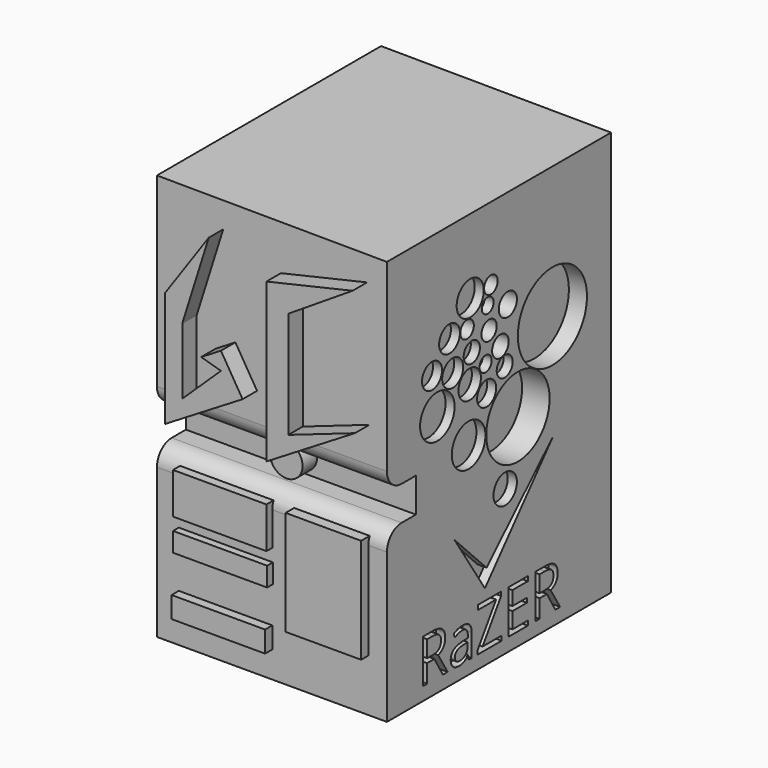
from build123d import *

# Parameters (mm, degrees)
F1_DEPTH      = 77.47
F3_DEPTH      = 5
F4_W          = 25.8451560512
F4_H          = 11.3645372912
F4_W_2        = 26.0284543037
F4_H_2        = 5.3156707436
F5_DEPTH      = 2
F6_R          = 2.3473696574
F7_DEPTH      = 10
F8_R          = 2.3473719846
F9_DEPTH      = 5
F10_R         = 2.6437582776
F11_DEPTH     = 5
F12_R         = 3.137573147
F13_DEPTH     = 5
F14_R         = 2.8690843811
F15_DEPTH     = 5
F16_R         = 11.9496313733
F17_DEPTH     = 5
F18_R         = 10.9566184267
F19_DEPTH     = 7.62
F20_W         = 59.5721621066
F20_H         = 108.5129901767
F21_DEPTH     = 0.5
F22_W         = 17.9633004591
F22_H         = 7.5152590871
F22_W_2       = 17.7800012752
F22_H_2       = 5.4989699274
F22_W_3       = 4.9490742385
F22_H_3       = 2.7494849637
F22_W_4       = 23.4622657299
F22_H_4       = 5.1323715597
F22_W_5       = 23.0956692249
F22_H_5       = 5.3156688809
F22_W_6       = 5.1323715597
F22_W_7       = 5.1323659718
F23_DEPTH     = 4
F24_TEXT_SIZE = 26.2153474792
F25_DEPTH     = 8.382
F26_R         = 6.3549509032
F27_DEPTH     = 6.604
F28_W         = 25.8451560512
F28_H         = 5.8655701578
F28_W_2       = 20.8960818127
F28_H_2       = 28.9612365887
F29_DEPTH     = 2.5
F30_R         = 3.6383810655
F30_R_2       = 3.8883576081
F30_R_3       = 3.3044699567
F30_R_4       = 2.0493435113
F30_R_5       = 2.8039346928
F30_R_6       = 2.0899281645
F30_R_7       = 5.8253336684
F30_R_8       = 5.967781049
F30_R_9       = 2.7494855225
F30_R_10      = 4.6839974373
F30_R_11      = 3.6012530141
F30_R_12      = 3.4584789248
F31_DEPTH     = 2.5
F32_W         = 18.5131970793
F32_H         = 58.8389690965
F33_DEPTH     = 1.5
F34_W         = 15.5804110691
F34_H         = 5.4989689961
F34_W_2       = 4.0325764567
F34_H_2       = 7.8818553593
F34_H_3       = 8.065154776
F34_W_3       = 4.4908244163
F34_W_4       = 15.2138136327
F34_H_4       = 5.6822672486
F35_DEPTH     = 5.588
F36_R         = 3.3044699309
F37_DEPTH     = 4.318
F38_W         = 63.6047441512
F38_H         = 9.4942739233
F39_DEPTH     = 10
F40_T1_DEPTH  = 18.9321648002
F40_T6_DEPTH  = 28.0447434634
F40_T11_DEPTH = 42.0278358877
F40_T16_DEPTH = 89.0047441512
F40_T21_DEPTH = 89.0047441512
F40_T26_DEPTH = 89.0047441512
F40_T32_DEPTH = 89.0047441512
F41_R         = 4.4746184375
F42_DEPTH     = 5
F43_R         = 4.0432169308
F44_DEPTH     = 2.54
F45_TEXT_SIZE = 16.8991896013
F46_DEPTH     = 2.5


# Not quite as in the source:
# - a fillet or chamfer that OpenCascade refuses, or shapes differently, is made with other operations: its cross-section is extruded or revolved along the edge and cut away or added
# - Text() gives the source's letters only with a copy of the font that has no kerning and outlines rounded to 1/6400 em; it was checked with that copy


with BuildPart() as f1:
    # F0 (on Front) → F1 (new body)
    with BuildSketch(Plane.XZ):
        Polygon((18.4215474874, 56.0894832015), (-45.1831966639, 56.4560852945), (-45.1831966639, -55.9061877429), (18.4215474874, -55.9061877429), align=None)
    extrude(amount=F1_DEPTH)

    # F2 (on face) → F3 (join)
    with BuildSketch(Plane.XZ.offset(77.47)):
        Polygon((-34.1852605343, 26.0284524411), (-26.8532987684, 49.3074245751), (-38.9510318637, 31.8940207362), (-38.9510318637, 0), (-17.5050515682, 13.0142262205), (-23.4882612947, 22.8738825479), (-28.9533808628, 19.5574427582), (-23.4882612947, 17.9632995278), (-34.1852605343, 7.6985568739), align=None)
        Polygon((-4.8574223183, 37.9428863525), (12.9225775599, 49.3074245751), (-10.9062884003, 43.808452785), (-10.9062884003, 0), (13.5728147639, 14.8548390824), (-4.8574223183, 8.4317522123), align=None)
    extrude(amount=F3_DEPTH)

    # F4 (on face) → F5 (join)
    with BuildSketch(Plane.XZ.offset(77.47)):
        with Locations((-26.2117530219, -18.1465991773)):
            Rectangle(F4_W, F4_H)
        with Locations((-26.1201038957, -29.9693820998)):
            Rectangle(F4_W_2, F4_H_2)
    extrude(amount=F5_DEPTH)

    # F6 (on face) → F7 (cut)
    with BuildSketch(Plane.YZ.offset(18.4215474874)):
        with Locations((-41.5361337364, 35.9265990555)):
            Circle(F6_R)
    extrude(amount=-F7_DEPTH, mode=Mode.SUBTRACT)

    # F8 (on face) → F9 (cut, symmetric)
    with BuildSketch(Plane.YZ.offset(18.4215474874)):
        with Locations((-49.7845895588, 28.4113399684)):
            Circle(F8_R)
    extrude(amount=F9_DEPTH, both=True, mode=Mode.SUBTRACT)

    # F10 (on face) → F11 (cut, symmetric)
    with BuildSketch(Plane.YZ.offset(18.4215474874)):
        with Locations((-42.1596653759, 25.0808000565)):
            Circle(F10_R)
    extrude(amount=F11_DEPTH, both=True, mode=Mode.SUBTRACT)

    # F12 (on face) → F13 (cut, symmetric)
    with BuildSketch(Plane.YZ.offset(18.4215474874)):
        with Locations((-35.6705673039, 28.7779401988)):
            Circle(F12_R)
    extrude(amount=F13_DEPTH, both=True, mode=Mode.SUBTRACT)

    # F14 (on face) → F15 (cut, symmetric)
    with BuildSketch(Plane.YZ.offset(18.4215474874)):
        with Locations((-38.2367521524, 19.6129903197)):
            Circle(F14_R)
    extrude(amount=F15_DEPTH, both=True, mode=Mode.SUBTRACT)

    # F16 (on face) → F17 (cut, symmetric)
    with BuildSketch(Plane.YZ.offset(18.4215474874)):
        with Locations((-20.2734526247, 19.6129903197)):
            Circle(F16_R)
    extrude(amount=F17_DEPTH, both=True, mode=Mode.SUBTRACT)

    # F18 (on face) → F19 (cut, symmetric)
    with BuildSketch(Plane.YZ.offset(18.4215474874)):
        with Locations((-32.1878865361, 0)):
            Circle(F18_R)
    extrude(amount=F19_DEPTH, both=True, mode=Mode.SUBTRACT)

    # F20 (on face) → F21 (cut, symmetric)
    with BuildSketch(Plane.XZ):
        with Locations((-13.5641237721, 0.1832991838)):
            Rectangle(F20_W, F20_H)
    extrude(amount=F21_DEPTH, both=True, mode=Mode.SUBTRACT)

    # F22 (on face) → F23 (cut, symmetric)
    with BuildSketch(Plane.XZ):
        with Locations((2.84113409, 43.9001061022)):
            Rectangle(F22_W, F22_H)
        with Locations((2.7494844981, 26.7616501078)):
            Rectangle(F22_W_2, F22_H_2)
        with Locations((-20.1628860086, 7.2403098457)):
            Rectangle(F22_W_3, F22_H_3)
        with Locations((-30.7025760412, -9.3482481316)):
            Rectangle(F22_W_4, F22_H_4)
        with Locations((-30.8858742937, -31.0691744089)):
            Rectangle(F22_W_5, F22_H_5)
        with Locations((-28.3196913078, 7.2403098457)):
            Rectangle(F22_W_6, F22_H_3)
        with Locations((-37.1180418879, 7.2403098457)):
            Rectangle(F22_W_7, F22_H_3)
    extrude(amount=F23_DEPTH, both=True, mode=Mode.SUBTRACT)

    # F24 (on face) → F25 (cut, symmetric)
    with BuildSketch(Plane(origin=(-45.1831966639, 0, 0), x_dir=(0, -1, 0), z_dir=(-1, 0, 0))):
        with Locations((0, 37.3868159599)):
            Text('RaZER', F24_TEXT_SIZE, font='Open Sans', text_align=(TextAlign.LEFT, TextAlign.BOTTOM))
    extrude(amount=F25_DEPTH, both=True, mode=Mode.SUBTRACT)

    # F26 (on face) → F27 (cut)
    with BuildSketch(Plane(origin=(-45.1831966639, 0, 0), x_dir=(0, -1, 0), z_dir=(-1, 0, 0))):
        with Locations((43.9190194011, 28.96123752)):
            Circle(F26_R)
        Polygon((22.6563382894, -27.8614442796), (56.2000535429, 33.1771150231), (22.4730409682, -14.8472161964), (7.6258247718, 3.849278437), align=None)
    extrude(amount=-F27_DEPTH, mode=Mode.SUBTRACT)

    # F28 (on face) → F29 (join)
    with BuildSketch(Plane.XZ.offset(77.47)):
        with Locations((-26.2117530219, -45.6414464861)):
            Rectangle(F28_W, F28_H)
        with Locations((2.84113409, -26.944948826)):
            Rectangle(F28_W_2, F28_H_2)
    extrude(amount=F29_DEPTH)

    # F30 (on face) → F31 (cut, symmetric)
    with BuildSketch(Plane.YZ.offset(18.4215474874)):
        with Locations((-54.7336600721, 19.7962895036)):
            Circle(F30_R)
        with Locations((-48.8680936396, 14.6639179438)):
            Circle(F30_R_2)
        with Locations((-43.0025272071, 10.0814439356)):
            Circle(F30_R_3)
        with Locations((-42.6359288394, 31.3441231847)):
            Circle(F30_R_4)
        with Locations((-48.1348969042, 22.1791770309)):
            Circle(F30_R_5)
        with Locations((-43.3691218495, 17.4134019762)):
            Circle(F30_R_6)
        with Locations((-49.2346920073, 0)):
            Circle(F30_R_7)
        with Locations((-60.049328953, 11.3645354286)):
            Circle(F30_R_8)
        with Locations((-36.770362407, 14.1140213236)):
            Circle(F30_R_9)
        with Locations((-48.6847944558, 35.5600006878)):
            Circle(F30_R_10)
        with Locations((-55.8334514499, 28.5946391523)):
            Circle(F30_R_11)
        with Locations((-61.8823207915, 21.9958759844)):
            Circle(F30_R_12)
    extrude(amount=F31_DEPTH, both=True, mode=Mode.SUBTRACT)

    # F32 (on face) → F33 (cut, symmetric)
    with BuildSketch(Plane.XZ):
        with Locations((2.7494840324, -11.8227833882)):
            Rectangle(F32_W, F32_H)
    extrude(amount=F33_DEPTH, both=True, mode=Mode.SUBTRACT)

    # F34 (on face) → F35 (cut, symmetric)
    with BuildSketch(Plane.XZ):
        with Locations((2.9327836819, 13.3808250539)):
            Rectangle(F34_W, F34_H)
        with Locations((8.7067009881, -0.6415463286)):
            Rectangle(F34_W_2, F34_H_2)
        with Locations((8.7067009881, -15.0305153802)):
            Rectangle(F34_W_2, F34_H_3)
        with Locations((-2.2454122081, -0.6415463286)):
            Rectangle(F34_W_3, F34_H_2)
        with Locations((-2.2454122081, -15.0305153802)):
            Rectangle(F34_W_3, F34_H_3)
        with Locations((3.1160824001, -28.3196922392)):
            Rectangle(F34_W_4, F34_H_4)
    extrude(amount=F35_DEPTH, both=True, mode=Mode.SUBTRACT)

    # F36 (on face) → F37 (cut)
    with BuildSketch(Plane.XZ):
        with Locations((-25.3869071603, 46.0080429912)):
            Circle(F36_R)
        Polygon((-23.3706198633, 29.3278358877), (-34.7351543605, 46.9245389104), (-22.454123944, 24.3787616491), (-16.9551540166, 35.376701504), align=None)
    extrude(amount=F37_DEPTH, mode=Mode.SUBTRACT)

    # F38 (on face) → F39 (cut)
    with BuildSketch(Plane.XZ.offset(77.47)):
        with Locations((-13.3808245882, -4.7471369617)):
            Rectangle(F38_W, F38_H)
    extrude(amount=-F39_DEPTH, mode=Mode.SUBTRACT)

    # F40: fillet of radius 5.08 on 4 edges, made by hand

    # F40_s2 → F40_t1 (cut)
    with BuildSketch(Plane.YZ.offset(-57.8831966639)):
        with BuildLine():
            ThreePointArc((-77.47, 5.08), (-75.9821024484, 1.4878975516), (-72.39, 0))
            Line((-72.39, 0), (-77.47, 0))
            Line((-77.47, 0), (-77.47, 5.08))
        make_face()
    extrude(amount=F40_T1_DEPTH, mode=Mode.SUBTRACT)


with BuildPart() as f40_tool4:
    # F40_s5 → F40_t6 (new body)
    with BuildSketch(Plane.YZ.offset(-10.9062884003)):
        with BuildLine():
            ThreePointArc((-77.47, 5.08), (-75.9821024484, 1.4878975516), (-72.39, 0))
            Line((-72.39, 0), (-77.47, 0))
            Line((-77.47, 0), (-77.47, 5.08))
        make_face()
    extrude(amount=-F40_T6_DEPTH)

    split(bisect_by=Plane(origin=(-10.4832955965, 0, 17.2752914375), x_dir=(0, 1, 0), z_dir=(0.5187874151, 0, -0.8549032799)), keep=Keep.TOP)


with BuildPart() as f1_1:
    add(f1.part)

    # F40_t3: cut F40_tool4
    add(f40_tool4.part, mode=Mode.SUBTRACT)


with BuildPart() as f40_tool9:
    # F40_s10 → F40_t11 (new body)
    with BuildSketch(Plane.YZ.offset(31.1215474874)):
        with BuildLine():
            ThreePointArc((-77.47, 5.08), (-75.9821024484, 1.4878975516), (-72.39, 0))
            Line((-72.39, 0), (-77.47, 0))
            Line((-77.47, 0), (-77.47, 5.08))
        make_face()
    extrude(amount=-F40_T11_DEPTH)

    split(bisect_by=Plane(origin=(-2.9353226266, 0, 4.8370813712), x_dir=(0, 1, 0), z_dir=(0.5187874151, 0, -0.8549032799)), keep=Keep.TOP)


with BuildPart() as f1_2:
    add(f1_1.part)

    # F40_t8: cut F40_tool9
    add(f40_tool9.part, mode=Mode.SUBTRACT)


with BuildPart() as f40_tool14:
    # F40_s15 → F40_t16 (new body)
    with BuildSketch(Plane.YZ.offset(-57.8831966639)):
        with BuildLine():
            ThreePointArc((-72.39, -9.4942739233), (-75.9821024484, -10.9821714749), (-77.47, -14.5742739233))
            Line((-77.47, -14.5742739233), (-77.47, -9.4942739233))
            Line((-77.47, -9.4942739233), (-72.39, -9.4942739233))
        make_face()
    extrude(amount=F40_T16_DEPTH)

    split(bisect_by=Plane.XY.offset(-12.4643305317), keep=Keep.TOP)


with BuildPart() as f1_3:
    add(f1_2.part)

    # F40_t13: cut F40_tool14
    add(f40_tool14.part, mode=Mode.SUBTRACT)


with BuildPart() as f40_tool19:
    # F40_s20 → F40_t21 (new body)
    with BuildSketch(Plane.YZ.offset(-57.8831966639)):
        with BuildLine():
            ThreePointArc((-72.39, -9.4942739233), (-75.9821024484, -10.9821714749), (-77.47, -14.5742739233))
            Line((-77.47, -14.5742739233), (-77.47, -9.4942739233))
            Line((-77.47, -9.4942739233), (-72.39, -9.4942739233))
        make_face()
    extrude(amount=F40_T21_DEPTH)

    split(bisect_by=Plane.YZ.offset(-39.1343310475), keep=Keep.BOTTOM)


with BuildPart() as f1_4:
    add(f1_3.part)

    # F40_t18: cut F40_tool19
    add(f40_tool19.part, mode=Mode.SUBTRACT)


with BuildPart() as f40_tool24:
    # F40_s25 → F40_t26 (new body)
    with BuildSketch(Plane.YZ.offset(-57.8831966639)):
        with BuildLine():
            ThreePointArc((-72.39, -9.4942739233), (-75.9821024484, -10.9821714749), (-77.47, -14.5742739233))
            Line((-77.47, -14.5742739233), (-77.47, -9.4942739233))
            Line((-77.47, -9.4942739233), (-72.39, -9.4942739233))
        make_face()
    extrude(amount=F40_T26_DEPTH)

    split(bisect_by=Plane.YZ.offset(-13.2891749963), keep=Keep.TOP)

    split(bisect_by=Plane.YZ.offset(-7.6069068164), keep=Keep.BOTTOM)


with BuildPart() as f1_5:
    add(f1_4.part)

    # F40_t23: cut F40_tool24
    add(f40_tool24.part, mode=Mode.SUBTRACT)


with BuildPart() as f40_tool30:
    # F40_s31 → F40_t32 (new body)
    with BuildSketch(Plane.YZ.offset(-57.8831966639)):
        with BuildLine():
            ThreePointArc((-72.39, -9.4942739233), (-75.9821024484, -10.9821714749), (-77.47, -14.5742739233))
            Line((-77.47, -14.5742739233), (-77.47, -9.4942739233))
            Line((-77.47, -9.4942739233), (-72.39, -9.4942739233))
        make_face()
    extrude(amount=F40_T32_DEPTH)

    split(bisect_by=Plane.YZ.offset(13.2891749963), keep=Keep.TOP)


with BuildPart() as f1_6:
    add(f1_5.part)

    # F40_t29: cut F40_tool30
    add(f40_tool30.part, mode=Mode.SUBTRACT)

    # F41 (on face) → F42 (join)
    with BuildSketch(Plane.XZ.offset(67.47)):
        with Locations((-13.3808245882, -4.5166932978)):
            Circle(F41_R)
    extrude(amount=F42_DEPTH)

    # F43 (on face) → F44 (cut, symmetric)
    with BuildSketch(Plane.YZ.offset(18.4215474874)):
        Polygon((-43.0478230119, -32.354272902), (-54.1091114283, -21.108629182), (-43.6008870602, -37.1474996209), (-19.9083060751, -9.5940933138), align=None)
        with Locations((-36.5954041481, -15.7623384148)):
            Circle(F43_R)
    extrude(amount=F44_DEPTH, both=True, mode=Mode.SUBTRACT)

    # F45 (on face) → F46 (cut, symmetric)
    with BuildSketch(Plane.YZ.offset(18.4215474874)):
        with Locations((-66.6452459991, -52.2645935416)):
            Text('RaZER', F45_TEXT_SIZE, font='Open Sans', text_align=(TextAlign.LEFT, TextAlign.BOTTOM))
    extrude(amount=F46_DEPTH, both=True, mode=Mode.SUBTRACT)


solid = f1_6.part
